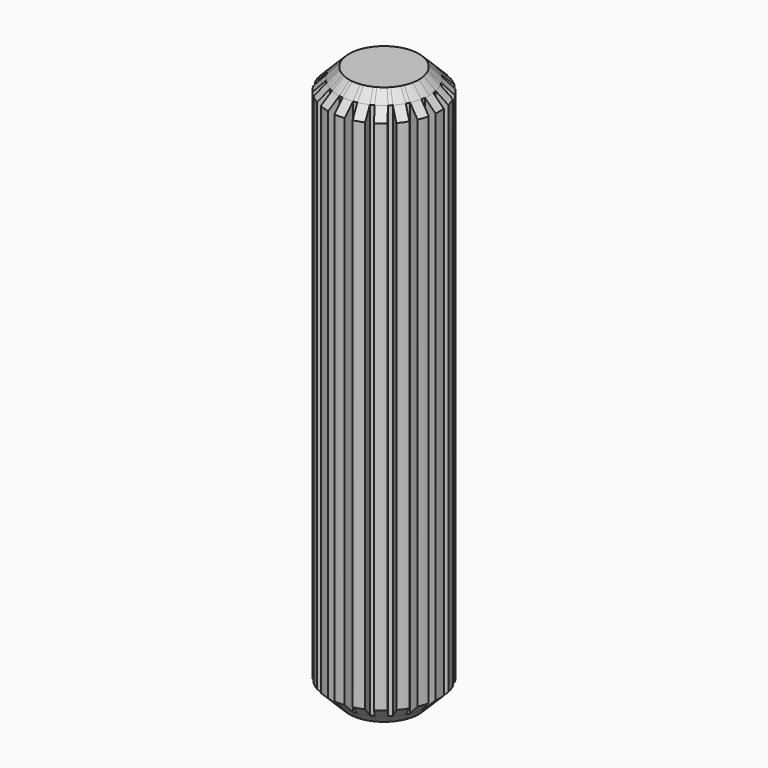
from build123d import *

# Parameters (mm, degrees)
F1_DEPTH = 20
F2_SIZE  = 0.75
F3_DEPTH = 19.25
F4_SIZE  = 0.74999
F5_COUNT = 20


# Not quite as in the source:
# - a fillet or chamfer is up to 0.001 mm smaller than in the source, because OpenCascade refuses the exact size


with BuildPart() as f1:
    # F0 (on Top) → F1 (new body, symmetric)
    with BuildSketch(Plane.XY):
        with BuildLine():
            ThreePointArc((3.25, 0), (2.4270609799, 2.1614520582), (0.375, 3.2282928925))
            Line((0.375, 3.2282928925), (0.375, 0))
            ThreePointArc((0.375, 0), (0, -0.375), (-0.375, 0))
            Line((-0.375, 0), (-0.375, 3.2282928925))
            ThreePointArc((-0.375, 3.2282928925), (-2.1614520582, -2.4270609799), (3.25, 0))
        make_face()
        with BuildLine():
            ThreePointArc((-0.375, 0), (0, -0.375), (0.375, 0))
            ThreePointArc((0.375, 0), (0, 0.375), (-0.375, 0))
        make_face()
        with BuildLine():
            Line((0.375, 0), (0.375, 3.2282928925))
            ThreePointArc((0.375, 3.2282928925), (0, 3.25), (-0.375, 3.2282928925))
            Line((-0.375, 3.2282928925), (-0.375, 0))
            ThreePointArc((-0.375, 0), (0, 0.375), (0.375, 0))
        make_face()
    extrude(amount=F1_DEPTH, both=True)

    # F2
    f2_edges = [f1.edges().sort_by_distance(p)[0] for p in [
        (-0.375, -3.228293, 20),
        (-0.375, -3.228293, -20),
    ]]
    chamfer(f2_edges, length=F2_SIZE)

    # F0 (on Top) → F3 (join, symmetric)
    with BuildSketch(Plane.XY):
        with BuildLine():
            Line((0.375, 3.2282928925), (0.375, 3.9823830805))
            ThreePointArc((0.375, 3.9823830805), (0, 4), (-0.375, 3.9823830805))
            Line((-0.375, 3.9823830805), (-0.375, 3.2282928925))
            ThreePointArc((-0.375, 3.2282928925), (0, 3.25), (0.375, 3.2282928925))
        make_face()
    extrude(amount=F3_DEPTH, both=True)

    # F4 (size 0.75 in the source; OpenCascade refuses exactly that, so slightly less here)
    f4_edges = [f1.edges().sort_by_distance(p)[0] for p in [
        (0, 4, 19.25),
        (0, 4, -19.25),
    ]]
    chamfer(f4_edges, length=F4_SIZE)

    # F5: F1 ×20 about axis
    f5_axis = Axis((0, 0, 0), (0, 0, 1))


with BuildPart() as f1_1:
    add(f1.part)
    for i in range(1, F5_COUNT):
        add(f1.part.rotate(f5_axis, i * 360 / F5_COUNT))


solid = f1_1.part
